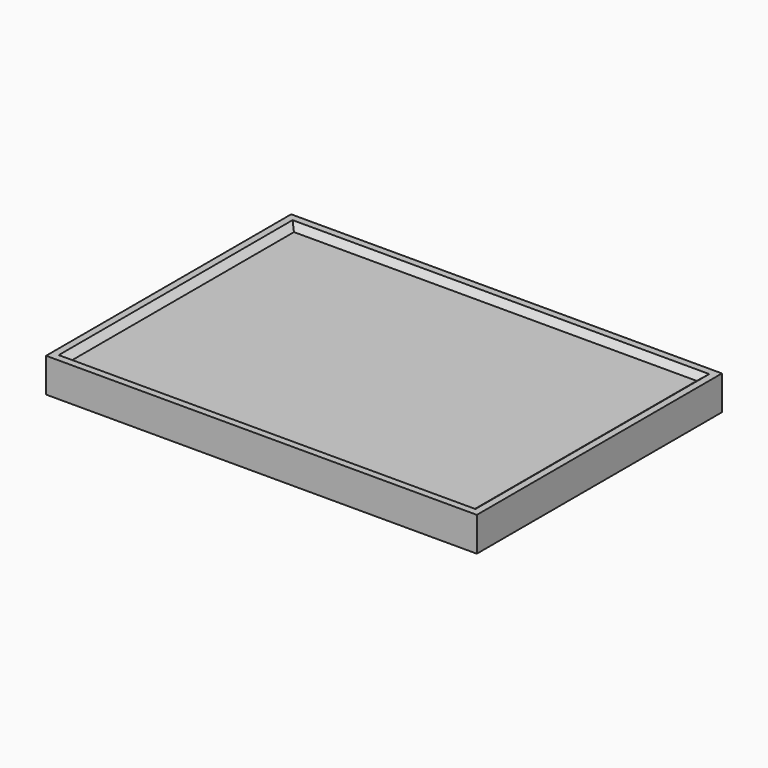
from build123d import *

# Parameters (mm, degrees)
F0_W         = 277
F0_H         = 197
F1_DEPTH     = 22
F2_W         = 268
F2_H         = 188
F3_DEPTH     = 3.5
F4_T4_DEPTH  = 188
F4_T9_DEPTH  = 268
F4_T14_DEPTH = 188
F4_T19_DEPTH = 268


# Not quite as in the source:
# - a fillet or chamfer that OpenCascade refuses, or shapes differently, is made with other operations: its cross-section is extruded or revolved along the edge and cut away or added


with BuildPart() as f1:
    # F0 (on Top) → F1 (new body)
    with BuildSketch(Plane.XY):
        Rectangle(F0_W, F0_H)
    extrude(amount=F1_DEPTH)

    # F2 (on face) → F3 (cut)
    with BuildSketch(Plane.XY.offset(22)):
        Rectangle(F2_W, F2_H)
    extrude(amount=-F3_DEPTH, mode=Mode.SUBTRACT)

    # F4: chamfer of 4.5 x 3.5157853193 on 4 edges, made by hand


with BuildPart() as f4_tool2:
    # F4_s3 → F4_t4 (new body)
    with BuildSketch(Plane.XZ.offset(94)):
        Polygon((134, 22.0157853193), (129.5, 18.5), (134, 18.5), align=None)
    extrude(amount=-F4_T4_DEPTH)

    split(bisect_by=Plane.XY.offset(22), keep=Keep.BOTTOM)


with BuildPart() as f1_1:
    add(f1.part)

    # F4_t1: union F4_tool2
    add(f4_tool2.part)


with BuildPart() as f4_tool7:
    # F4_s8 → F4_t9 (new body)
    with BuildSketch(Plane.YZ.offset(134)):
        Polygon((94, 22.0157853193), (89.5, 18.5), (94, 18.5), align=None)
    extrude(amount=-F4_T9_DEPTH)

    split(bisect_by=Plane.XY.offset(22), keep=Keep.BOTTOM)


with BuildPart() as f1_2:
    add(f1_1.part)

    # F4_t6: union F4_tool7
    add(f4_tool7.part)


with BuildPart() as f4_tool12:
    # F4_s13 → F4_t14 (new body)
    with BuildSketch(Plane.XZ.offset(-94)):
        Polygon((-134, 22.0157853193), (-129.5, 18.5), (-134, 18.5), align=None)
    extrude(amount=F4_T14_DEPTH)

    split(bisect_by=Plane.XY.offset(22), keep=Keep.BOTTOM)


with BuildPart() as f1_3:
    add(f1_2.part)

    # F4_t11: union F4_tool12
    add(f4_tool12.part)


with BuildPart() as f4_tool17:
    # F4_s18 → F4_t19 (new body)
    with BuildSketch(Plane.YZ.offset(-134)):
        Polygon((-94, 22.0157853193), (-89.5, 18.5), (-94, 18.5), align=None)
    extrude(amount=F4_T19_DEPTH)

    split(bisect_by=Plane.XY.offset(22), keep=Keep.BOTTOM)


with BuildPart() as f1_4:
    add(f1_3.part)

    # F4_t16: union F4_tool17
    add(f4_tool17.part)


solid = f1_4.part
